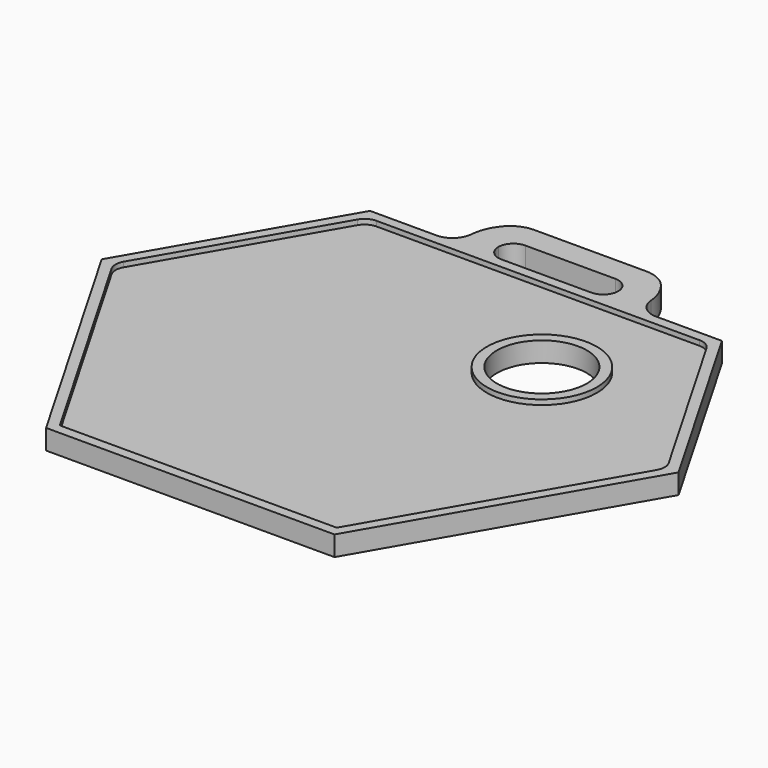
from build123d import *

# Parameters (mm, degrees)
F0_R     = 4.5
F0_W     = 12
F0_H     = 3
F1_DEPTH = 2
F2_R     = 5.5
F3_DEPTH = 0.5
F5_R     = 1.49999
F7_DEPTH = 25
F8_R     = 3


# Not quite as in the source:
# - a fillet or chamfer is up to 0.001 mm smaller than in the source, because OpenCascade refuses the exact size


with BuildPart() as f1:
    # F0 (on Top) → F1 (new body)
    with BuildSketch(Plane.XY):
        Polygon((14.4337567297, -25), (28.8675134595, 0), (14.4337567297, 25), (-14.4337567297, 25), (-28.8675134595, 0), (-14.4337567297, -25), align=None)
        with Locations((9.37942788, 7.2647714987)):
            Circle(F0_R, mode=Mode.SUBTRACT)
        with Locations((0.0337567297, 21)):
            Rectangle(F0_W, F0_H, mode=Mode.SUBTRACT)
    extrude(amount=F1_DEPTH)

    # F2 (on face) → F3 (cut)
    with BuildSketch(Plane.XY.offset(2)):
        Polygon((-13.8564064606, -24), (13.8564064606, -24), (27.7128129211, 0), (17.0318329411, 18.5), (-17.0318329411, 18.5), (-27.7128129211, 0), align=None)
        with Locations((9.37942788, 7.2647714987)):
            Circle(F2_R, mode=Mode.SUBTRACT)
    extrude(amount=-F3_DEPTH, mode=Mode.SUBTRACT)

    # F5 (radius 1.5 in the source; OpenCascade refuses exactly that, so slightly less here)
    f5_edges = [f1.edges().sort_by_distance(p)[0] for p in [
        (-5.966243, 19.5, 1),
        (6.033757, 19.5, 1),
        (6.033757, 22.5, 1),
        (-5.966243, 22.5, 1),
        (-17.031833, 18.5, 1.75),
        (-27.712813, 0, 1.75),
        (17.031833, 18.5, 1.75),
        (27.712813, 0, 1.75),
    ]]
    fillet(f5_edges, radius=F5_R)

    # F6 (on face) → F7 (cut)
    with BuildSketch(Plane.XY.offset(2)):
        with BuildLine():
            Line((-4.4662432703, 25.5), (4.5337567297, 25.5))
            ThreePointArc((4.5337567297, 25.5), (7.5909047219, 24.3020972357), (9.0204233671, 21.3461538462))
            ThreePointArc((9.0204233671, 21.3461538462), (9.6557649872, 20.0324012286), (11.0144974281, 19.5))
            Line((11.0144974281, 19.5), (21.36195996, 19.5))
            Line((21.36195996, 19.5), (25.703800239, 29.2692627907))
            Line((25.703800239, 29.2692627907), (-20.3538952839, 30.2788760662))
            Line((-20.3538952839, 30.2788760662), (-17.6091832103, 19.5))
            Line((-17.6091832103, 19.5), (-10.9469839687, 19.5))
            ThreePointArc((-10.9469839687, 19.5), (-9.5882515277, 20.0324012286), (-8.9529099076, 21.3461538462))
            ThreePointArc((-8.9529099076, 21.3461538462), (-7.5233912624, 24.3020972357), (-4.4662432703, 25.5))
        make_face()
    extrude(amount=-F7_DEPTH, mode=Mode.SUBTRACT)

    # F8
    f8_edges = [f1.edges().sort_by_distance(p)[0] for p in [
        (-6.527796, 25, 1),
        (6.59531, 25, 1),
    ]]
    fillet(f8_edges, radius=F8_R)


solid = f1.part
